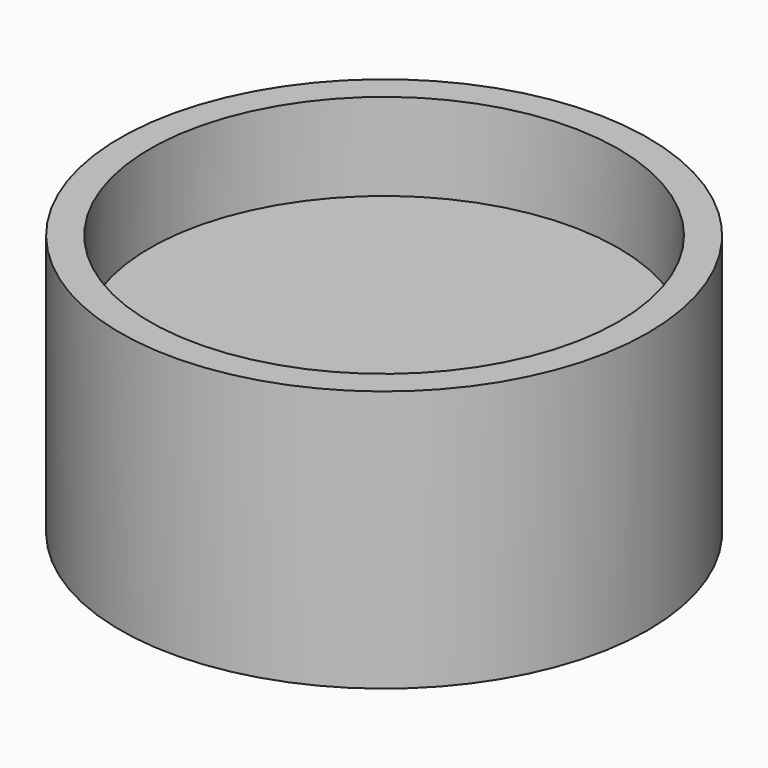
from build123d import *

# Parameters (mm, degrees)
F0_R         = 75.6647788215
F0_R_2       = 67.1352595914
F1_DEPTH     = 25
F2_DEPTH     = 25
F1_FACE_R    = 75.6647788215
F1_FACE_R_2  = 67.1352595914
F1_FACE1_R   = 75.6647788215
F1_FACE1_R_2 = 67.1352595914
F3_R         = 75.5867204447
F3_R_2       = 67.1352595914
F4_DEPTH     = 50


with BuildPart() as f1:
    # F0 (on Top) → F1 (new body)
    with BuildSketch(Plane.XY):
        Circle(F0_R)
        Circle(F0_R_2, mode=Mode.SUBTRACT)
    extrude(amount=F1_DEPTH)

    # F0 (on Top) → F2 (join)
    with BuildSketch(Plane.XY):
        Circle(F0_R)
        Circle(F0_R_2, mode=Mode.SUBTRACT)
    extrude(amount=F2_DEPTH)

    # F1_face (on face) + F1_face1 (on face) + F3 (on face) → F4 (join)
    with BuildSketch(Plane(origin=(0, 0, 0), x_dir=(1, 0, 0), z_dir=(0, 0, -1))):
        Circle(F1_FACE_R)
        Circle(F1_FACE_R_2, mode=Mode.SUBTRACT)
    with BuildSketch(Plane.XY.offset(25)):
        Circle(F1_FACE1_R)
        Circle(F1_FACE1_R_2, mode=Mode.SUBTRACT)
    with BuildSketch(Plane(origin=(0, 0, 0), x_dir=(1, 0, 0), z_dir=(0, 0, -1))):
        Circle(F3_R)
        Circle(F3_R_2, mode=Mode.SUBTRACT)
        Circle(F3_R_2)
    extrude(amount=F4_DEPTH, dir=(0, 0, -1))


solid = f1.part
